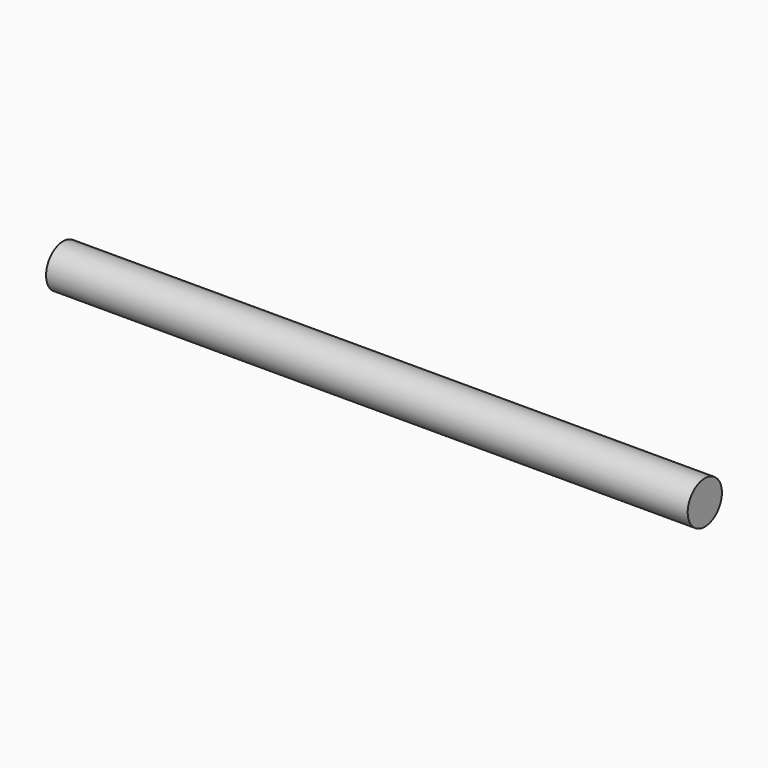
from build123d import *

# Parameters (mm, degrees)
F0_R     = 5
F1_DEPTH = 150


with BuildPart() as f1:
    # F0 (on Right) → F1 (new body)
    with BuildSketch(Plane.YZ):
        Circle(F0_R)
    extrude(amount=F1_DEPTH)


solid = f1.part
